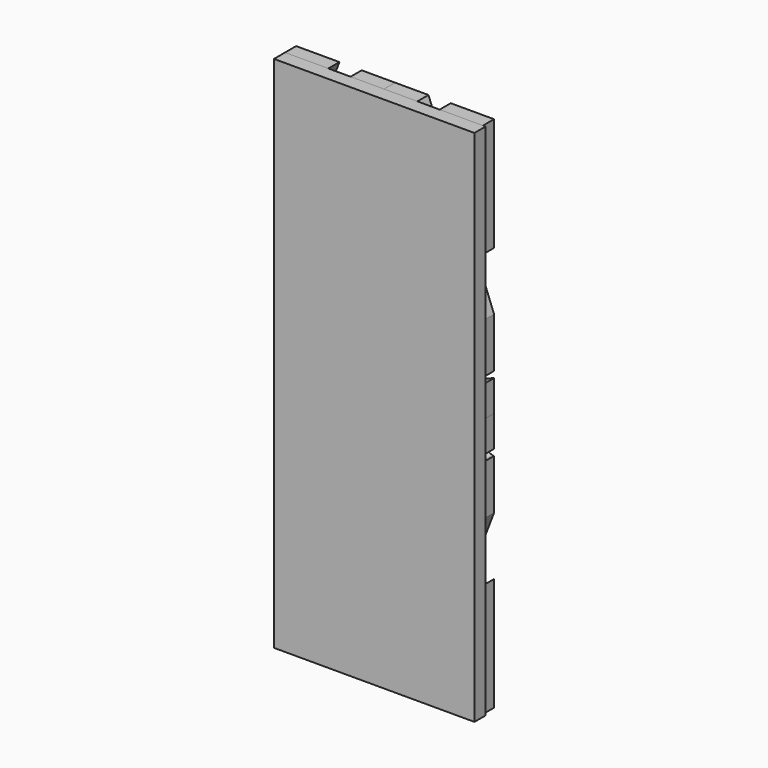
from build123d import *

# Parameters (mm, degrees)
F1_DEPTH = 2.54
F2_W     = 36.7250956763
F2_H     = 94.9781656687
F3_DEPTH = 2.54


with BuildPart() as f1:
    # F0 (on Front) → F1 (new body)
    with BuildSketch(Plane.XZ):
        Polygon((-10.1961911618, 47.455956084), (-18.1265615095, 47.455956084), (-18.1265615095, 26.6939761161), align=None)
    extrude(amount=F1_DEPTH)


with BuildPart() as f1b:
    # F0 (on Front) → F1, piece 2 (new body)
    with BuildSketch(Plane.XZ):
        Polygon((-3.3987303873, 47.455956084), (-6.1177146971, 47.455956084), (-18.1265615095, 16.0163856696), (-18.1265615095, 8.8979920387), align=None)
        with BuildLine():
            Line((0, 47.455956084), (-3.3987303873, 47.455956084))
            Line((-3.3987303873, 47.455956084), (-18.1265615095, 8.8979920387))
            Line((-18.1265615095, 8.8979920387), (-18.1265615095, 6.8514491871))
            ThreePointArc((-18.1265615095, 6.8514491871), (-17.9774288105, 6.8556010302), (-17.8323030506, 6.8210132649))
            Line((-17.8323030506, 6.8210132649), (-15.815424917, 6.0506344007))
            Line((-15.815424917, 6.0506344007), (-14.6774796667, 9.029813866))
            Line((-14.6774796667, 9.029813866), (-16.6943578003, 9.8001927301))
            ThreePointArc((-16.6943578003, 9.8001927301), (-17.0243134892, 10.5379960531), (-16.2865101663, 10.867951742))
            Line((-16.2865101663, 10.867951742), (-14.2696320327, 10.0975728779))
            Line((-14.2696320327, 10.0975728779), (-13.1316867824, 13.0767523431))
            Line((-13.1316867824, 13.0767523431), (-15.148564916, 13.8471312073))
            ThreePointArc((-15.148564916, 13.8471312073), (-15.478520605, 14.5849345302), (-14.740717282, 14.9148902192))
            Line((-14.740717282, 14.9148902192), (-12.7238391485, 14.144511355))
            Line((-12.7238391485, 14.144511355), (-11.5858938981, 17.1236908203))
            Line((-11.5858938981, 17.1236908203), (-13.6027720317, 17.8940696845))
            ThreePointArc((-13.6027720317, 17.8940696845), (-13.9327277207, 18.6318730074), (-13.1949243977, 18.9618286963))
            Line((-13.1949243977, 18.9618286963), (-11.1780462642, 18.1914498322))
            Line((-11.1780462642, 18.1914498322), (-10.0401010139, 21.1706292975))
            Line((-10.0401010139, 21.1706292975), (-12.0569791474, 21.9410081616))
            ThreePointArc((-12.0569791474, 21.9410081616), (-12.3869348364, 22.6788114845), (-11.6491315135, 23.0087671735))
            Line((-11.6491315135, 23.0087671735), (-9.6322533799, 22.2383883093))
            Line((-9.6322533799, 22.2383883093), (-9.0632807547, 23.727978042))
            Line((-9.0632807547, 23.727978042), (-8.4943081296, 25.2175677746))
            Line((-8.4943081296, 25.2175677746), (-10.5111862631, 25.9879466388))
            ThreePointArc((-10.5111862631, 25.9879466388), (-10.8411419521, 26.7257499617), (-10.1033386292, 27.0557056507))
            Line((-10.1033386292, 27.0557056507), (-8.0864604956, 26.2853267865))
            Line((-8.0864604956, 26.2853267865), (-6.9485152453, 29.2645062518))
            Line((-6.9485152453, 29.2645062518), (-8.9653933789, 30.0348851159))
            ThreePointArc((-8.9653933789, 30.0348851159), (-9.2953490678, 30.7726884389), (-8.5575457449, 31.1026441278))
            Line((-8.5575457449, 31.1026441278), (-6.5406676113, 30.3322652637))
            Line((-6.5406676113, 30.3322652637), (-5.402722361, 33.3114447289))
            Line((-5.402722361, 33.3114447289), (-7.4196004946, 34.0818235931))
            ThreePointArc((-7.4196004946, 34.0818235931), (-7.7495561835, 34.819626916), (-7.0117528606, 35.149582605))
            Line((-7.0117528606, 35.149582605), (-4.9948747271, 34.3792037408))
            Line((-4.9948747271, 34.3792037408), (-3.8569294767, 37.3583832061))
            Line((-3.8569294767, 37.3583832061), (-5.8738076103, 38.1287620703))
            ThreePointArc((-5.8738076103, 38.1287620703), (-6.2037632993, 38.8665653932), (-5.4659599763, 39.1965210821))
            Line((-5.4659599763, 39.1965210821), (-3.4490818428, 38.426142218))
            Line((-3.4490818428, 38.426142218), (-2.3111365925, 41.4053216833))
            Line((-2.3111365925, 41.4053216833), (-4.328014726, 42.1757005474))
            ThreePointArc((-4.328014726, 42.1757005474), (-4.657970415, 42.9135038703), (-3.9201670921, 43.2434595593))
            Line((-3.9201670921, 43.2434595593), (-1.9032889585, 42.4730806951))
            Line((-1.9032889585, 42.4730806951), (0, 47.455956084))
        make_face()
    extrude(amount=F1_DEPTH)


with BuildPart() as f1c:
    # F0 (on Front) → F1, piece 3 (new body)
    with BuildSketch(Plane.XZ):
        with BuildLine():
            Line((3.3987303873, 47.455956084), (0, 47.455956084))
            Line((0, 47.455956084), (1.9032889585, 42.4730806951))
            Line((1.9032889585, 42.4730806951), (3.9201670921, 43.2434595593))
            ThreePointArc((3.9201670921, 43.2434595593), (4.657970415, 42.9135038703), (4.328014726, 42.1757005474))
            Line((4.328014726, 42.1757005474), (2.3111365925, 41.4053216833))
            Line((2.3111365925, 41.4053216833), (3.4490818428, 38.426142218))
            Line((3.4490818428, 38.426142218), (5.4659599763, 39.1965210821))
            ThreePointArc((5.4659599763, 39.1965210821), (6.2037632993, 38.8665653932), (5.8738076103, 38.1287620703))
            Line((5.8738076103, 38.1287620703), (3.8569294767, 37.3583832061))
            Line((3.8569294767, 37.3583832061), (4.9948747271, 34.3792037408))
            Line((4.9948747271, 34.3792037408), (7.0117528606, 35.149582605))
            ThreePointArc((7.0117528606, 35.149582605), (7.7495561835, 34.819626916), (7.4196004946, 34.0818235931))
            Line((7.4196004946, 34.0818235931), (5.402722361, 33.3114447289))
            Line((5.402722361, 33.3114447289), (6.5406676113, 30.3322652637))
            Line((6.5406676113, 30.3322652637), (8.5575457449, 31.1026441278))
            ThreePointArc((8.5575457449, 31.1026441278), (9.2953490678, 30.7726884389), (8.9653933789, 30.0348851159))
            Line((8.9653933789, 30.0348851159), (6.9485152453, 29.2645062518))
            Line((6.9485152453, 29.2645062518), (8.0864604956, 26.2853267865))
            Line((8.0864604956, 26.2853267865), (10.1033386292, 27.0557056507))
            ThreePointArc((10.1033386292, 27.0557056507), (10.8411419521, 26.7257499617), (10.5111862631, 25.9879466388))
            Line((10.5111862631, 25.9879466388), (8.4943081296, 25.2175677746))
            Line((8.4943081296, 25.2175677746), (9.6322533799, 22.2383883093))
            Line((9.6322533799, 22.2383883093), (11.6491315135, 23.0087671735))
            ThreePointArc((11.6491315135, 23.0087671735), (12.3869348364, 22.6788114845), (12.0569791474, 21.9410081616))
            Line((12.0569791474, 21.9410081616), (10.0401010139, 21.1706292975))
            Line((10.0401010139, 21.1706292975), (11.1780462642, 18.1914498322))
            Line((11.1780462642, 18.1914498322), (13.1949243977, 18.9618286963))
            ThreePointArc((13.1949243977, 18.9618286963), (13.9327277207, 18.6318730074), (13.6027720317, 17.8940696845))
            Line((13.6027720317, 17.8940696845), (11.5858938981, 17.1236908203))
            Line((11.5858938981, 17.1236908203), (12.7238391485, 14.144511355))
            Line((12.7238391485, 14.144511355), (14.740717282, 14.9148902192))
            ThreePointArc((14.740717282, 14.9148902192), (15.478520605, 14.5849345302), (15.148564916, 13.8471312073))
            Line((15.148564916, 13.8471312073), (13.1316867824, 13.0767523431))
            Line((13.1316867824, 13.0767523431), (14.2696320327, 10.0975728779))
            Line((14.2696320327, 10.0975728779), (16.2865101663, 10.867951742))
            ThreePointArc((16.2865101663, 10.867951742), (17.0243134892, 10.5379960531), (16.6943578003, 9.8001927301))
            Line((16.6943578003, 9.8001927301), (14.6774796667, 9.029813866))
            Line((14.6774796667, 9.029813866), (15.815424917, 6.0506344007))
            Line((15.815424917, 6.0506344007), (17.8323030506, 6.8210132649))
            ThreePointArc((17.8323030506, 6.8210132649), (17.9774288105, 6.8556010302), (18.1265615095, 6.8514491871))
            Line((18.1265615095, 6.8514491871), (18.1265615095, 8.8979920387))
            Line((18.1265615095, 8.8979920387), (3.3987303873, 47.455956084))
        make_face()
        Polygon((6.1177146971, 47.455956084), (3.3987303873, 47.455956084), (18.1265615095, 8.8979920387), (18.1265615095, 16.0163856696), align=None)
    extrude(amount=F1_DEPTH)


with BuildPart() as f1d:
    # F0 (on Front) → F1, piece 4 (new body)
    with BuildSketch(Plane.XZ):
        Polygon((-16.223272551, 4.9828753888), (-18.1265615095, 5.7098670506), (-18.1265615095, 0), align=None)
    extrude(amount=F1_DEPTH)


with BuildPart() as f1e:
    # F0 (on Front) → F1, piece 5 (new body)
    with BuildSketch(Plane.XZ):
        Polygon((18.1265615095, 47.455956084), (10.1961911618, 47.455956084), (18.1265615095, 26.6939761161), align=None)
    extrude(amount=F1_DEPTH)


with BuildPart() as f1f:
    # F0 (on Front) → F1, piece 6 (new body)
    with BuildSketch(Plane.XZ):
        Polygon((-16.223272551, -4.9828753888), (-18.1265615095, 0), (-18.1265615095, -5.7098670506), align=None)
    extrude(amount=F1_DEPTH)


with BuildPart() as f1g:
    # F0 (on Front) → F1, piece 7 (new body)
    with BuildSketch(Plane.XZ):
        Polygon((18.1265615095, 0), (18.1265615095, 5.7098670506), (16.223272551, 4.9828753888), align=None)
    extrude(amount=F1_DEPTH)


with BuildPart() as f1h:
    # F0 (on Front) → F1, piece 8 (new body)
    with BuildSketch(Plane.XZ):
        Polygon((18.1265615095, -5.7098670506), (18.1265615095, 0), (16.223272551, -4.9828753888), align=None)
    extrude(amount=F1_DEPTH)


with BuildPart() as f1i:
    # F0 (on Front) → F1, piece 9 (new body)
    with BuildSketch(Plane.XZ):
        with BuildLine():
            ThreePointArc((-17.8323030506, -6.8210132649), (-17.9774288105, -6.8556010302), (-18.1265615095, -6.8514491871))
            Line((-18.1265615095, -6.8514491871), (-18.1265615095, -8.8979920387))
            Line((-18.1265615095, -8.8979920387), (-3.3987303873, -47.455956084))
            Line((-3.3987303873, -47.455956084), (0, -47.455956084))
            Line((0, -47.455956084), (-1.9032889585, -42.4730806951))
            Line((-1.9032889585, -42.4730806951), (-3.9201670921, -43.2434595593))
            ThreePointArc((-3.9201670921, -43.2434595593), (-4.657970415, -42.9135038703), (-4.328014726, -42.1757005474))
            Line((-4.328014726, -42.1757005474), (-2.3111365925, -41.4053216833))
            Line((-2.3111365925, -41.4053216833), (-3.4490818428, -38.426142218))
            Line((-3.4490818428, -38.426142218), (-5.4659599763, -39.1965210821))
            ThreePointArc((-5.4659599763, -39.1965210821), (-6.2037632993, -38.8665653932), (-5.8738076103, -38.1287620703))
            Line((-5.8738076103, -38.1287620703), (-3.8569294767, -37.3583832061))
            Line((-3.8569294767, -37.3583832061), (-4.9948747271, -34.3792037408))
            Line((-4.9948747271, -34.3792037408), (-7.0117528606, -35.149582605))
            ThreePointArc((-7.0117528606, -35.149582605), (-7.7495561835, -34.819626916), (-7.4196004946, -34.0818235931))
            Line((-7.4196004946, -34.0818235931), (-5.402722361, -33.3114447289))
            Line((-5.402722361, -33.3114447289), (-6.5406676113, -30.3322652637))
            Line((-6.5406676113, -30.3322652637), (-8.5575457449, -31.1026441278))
            ThreePointArc((-8.5575457449, -31.1026441278), (-9.2953490678, -30.7726884389), (-8.9653933789, -30.0348851159))
            Line((-8.9653933789, -30.0348851159), (-6.9485152453, -29.2645062518))
            Line((-6.9485152453, -29.2645062518), (-8.0864604956, -26.2853267865))
            Line((-8.0864604956, -26.2853267865), (-10.1033386292, -27.0557056507))
            ThreePointArc((-10.1033386292, -27.0557056507), (-10.8411419521, -26.7257499617), (-10.5111862631, -25.9879466388))
            Line((-10.5111862631, -25.9879466388), (-8.4943081296, -25.2175677746))
            Line((-8.4943081296, -25.2175677746), (-9.6322533799, -22.2383883093))
            Line((-9.6322533799, -22.2383883093), (-11.6491315135, -23.0087671735))
            ThreePointArc((-11.6491315135, -23.0087671735), (-12.3869348364, -22.6788114845), (-12.0569791474, -21.9410081616))
            Line((-12.0569791474, -21.9410081616), (-10.0401010139, -21.1706292975))
            Line((-10.0401010139, -21.1706292975), (-11.1780462642, -18.1914498322))
            Line((-11.1780462642, -18.1914498322), (-13.1949243977, -18.9618286963))
            ThreePointArc((-13.1949243977, -18.9618286963), (-13.9327277207, -18.6318730074), (-13.6027720317, -17.8940696845))
            Line((-13.6027720317, -17.8940696845), (-11.5858938981, -17.1236908203))
            Line((-11.5858938981, -17.1236908203), (-12.7238391485, -14.144511355))
            Line((-12.7238391485, -14.144511355), (-14.740717282, -14.9148902192))
            ThreePointArc((-14.740717282, -14.9148902192), (-15.478520605, -14.5849345302), (-15.148564916, -13.8471312073))
            Line((-15.148564916, -13.8471312073), (-13.1316867824, -13.0767523431))
            Line((-13.1316867824, -13.0767523431), (-14.2696320327, -10.0975728779))
            Line((-14.2696320327, -10.0975728779), (-16.2865101663, -10.867951742))
            ThreePointArc((-16.2865101663, -10.867951742), (-17.0243134892, -10.5379960531), (-16.6943578003, -9.8001927301))
            Line((-16.6943578003, -9.8001927301), (-14.6774796667, -9.029813866))
            Line((-14.6774796667, -9.029813866), (-15.815424917, -6.0506344007))
            Line((-15.815424917, -6.0506344007), (-17.8323030506, -6.8210132649))
        make_face()
        Polygon((-3.3987303873, -47.455956084), (-18.1265615095, -8.8979920387), (-18.1265615095, -16.0163856696), (-6.1177146971, -47.455956084), align=None)
    extrude(amount=F1_DEPTH)


with BuildPart() as f1j:
    # F0 (on Front) → F1, piece 10 (new body)
    with BuildSketch(Plane.XZ):
        with BuildLine():
            Line((18.1265615095, -8.8979920387), (18.1265615095, -6.8514491871))
            ThreePointArc((18.1265615095, -6.8514491871), (17.9774288105, -6.8556010302), (17.8323030506, -6.8210132649))
            Line((17.8323030506, -6.8210132649), (15.815424917, -6.0506344007))
            Line((15.815424917, -6.0506344007), (14.6774796667, -9.029813866))
            Line((14.6774796667, -9.029813866), (16.6943578003, -9.8001927301))
            ThreePointArc((16.6943578003, -9.8001927301), (17.0243134892, -10.5379960531), (16.2865101663, -10.867951742))
            Line((16.2865101663, -10.867951742), (14.2696320327, -10.0975728779))
            Line((14.2696320327, -10.0975728779), (13.1316867824, -13.0767523431))
            Line((13.1316867824, -13.0767523431), (15.148564916, -13.8471312073))
            ThreePointArc((15.148564916, -13.8471312073), (15.478520605, -14.5849345302), (14.740717282, -14.9148902192))
            Line((14.740717282, -14.9148902192), (12.7238391485, -14.144511355))
            Line((12.7238391485, -14.144511355), (11.5858938981, -17.1236908203))
            Line((11.5858938981, -17.1236908203), (13.6027720317, -17.8940696845))
            ThreePointArc((13.6027720317, -17.8940696845), (13.9327277207, -18.6318730074), (13.1949243977, -18.9618286963))
            Line((13.1949243977, -18.9618286963), (11.1780462642, -18.1914498322))
            Line((11.1780462642, -18.1914498322), (10.0401010139, -21.1706292975))
            Line((10.0401010139, -21.1706292975), (12.0569791474, -21.9410081616))
            ThreePointArc((12.0569791474, -21.9410081616), (12.3869348364, -22.6788114845), (11.6491315135, -23.0087671735))
            Line((11.6491315135, -23.0087671735), (9.6322533799, -22.2383883093))
            Line((9.6322533799, -22.2383883093), (8.4943081296, -25.2175677746))
            Line((8.4943081296, -25.2175677746), (10.5111862631, -25.9879466388))
            ThreePointArc((10.5111862631, -25.9879466388), (10.8411419521, -26.7257499617), (10.1033386292, -27.0557056507))
            Line((10.1033386292, -27.0557056507), (8.0864604956, -26.2853267865))
            Line((8.0864604956, -26.2853267865), (6.9485152453, -29.2645062518))
            Line((6.9485152453, -29.2645062518), (8.9653933789, -30.0348851159))
            ThreePointArc((8.9653933789, -30.0348851159), (9.2953490678, -30.7726884389), (8.5575457449, -31.1026441278))
            Line((8.5575457449, -31.1026441278), (6.5406676113, -30.3322652637))
            Line((6.5406676113, -30.3322652637), (5.402722361, -33.3114447289))
            Line((5.402722361, -33.3114447289), (7.4196004946, -34.0818235931))
            ThreePointArc((7.4196004946, -34.0818235931), (7.7495561835, -34.819626916), (7.0117528606, -35.149582605))
            Line((7.0117528606, -35.149582605), (4.9948747271, -34.3792037408))
            Line((4.9948747271, -34.3792037408), (3.8569294767, -37.3583832061))
            Line((3.8569294767, -37.3583832061), (5.8738076103, -38.1287620703))
            ThreePointArc((5.8738076103, -38.1287620703), (6.2037632993, -38.8665653932), (5.4659599763, -39.1965210821))
            Line((5.4659599763, -39.1965210821), (3.4490818428, -38.426142218))
            Line((3.4490818428, -38.426142218), (2.3111365925, -41.4053216833))
            Line((2.3111365925, -41.4053216833), (4.328014726, -42.1757005474))
            ThreePointArc((4.328014726, -42.1757005474), (4.657970415, -42.9135038703), (3.9201670921, -43.2434595593))
            Line((3.9201670921, -43.2434595593), (1.9032889585, -42.4730806951))
            Line((1.9032889585, -42.4730806951), (0, -47.455956084))
            Line((0, -47.455956084), (3.3987303873, -47.455956084))
            Line((3.3987303873, -47.455956084), (18.1265615095, -8.8979920387))
        make_face()
        Polygon((18.1265615095, -16.0163856696), (18.1265615095, -8.8979920387), (3.3987303873, -47.455956084), (6.1177146971, -47.455956084), align=None)
    extrude(amount=F1_DEPTH)


with BuildPart() as f1k:
    # F0 (on Front) → F1, piece 11 (new body)
    with BuildSketch(Plane.XZ):
        Polygon((-10.1961911618, -47.455956084), (-18.1265615095, -26.6939761161), (-18.1265615095, -47.455956084), align=None)
    extrude(amount=F1_DEPTH)


with BuildPart() as f1l:
    # F0 (on Front) → F1, piece 12 (new body)
    with BuildSketch(Plane.XZ):
        Polygon((18.1265615095, -47.455956084), (18.1265615095, -26.6939761161), (10.1961911618, -47.455956084), align=None)
    extrude(amount=F1_DEPTH)


with BuildPart() as f1m:
    # F0 (on Front) → F1, piece 13 (new body)
    with BuildSketch(Plane.XZ):
        with BuildLine():
            Line((0.3851894321, 28.6515334857), (0, 29.6599725525))
            Line((0, 29.6599725525), (-0.3851894321, 28.6515334857))
            Line((-0.3851894321, 28.6515334857), (-2.4020675656, 29.4219123498))
            ThreePointArc((-2.4020675656, 29.4219123498), (-3.1398708886, 29.0919566609), (-2.8099151996, 28.354153338))
            Line((-2.8099151996, 28.354153338), (-0.793037066, 27.5837744738))
            Line((-0.793037066, 27.5837744738), (-1.8353143528, 24.855056999))
            Line((-1.8353143528, 24.855056999), (-3.8521924864, 25.6254358631))
            ThreePointArc((-3.8521924864, 25.6254358631), (-4.5899958093, 25.2954801742), (-4.2600401204, 24.5576768512))
            Line((-4.2600401204, 24.5576768512), (-2.2431619868, 23.7872979871))
            Line((-2.2431619868, 23.7872979871), (-3.2854392736, 21.0585805123))
            Line((-3.2854392736, 21.0585805123), (-5.3023174072, 21.8289593764))
            ThreePointArc((-5.3023174072, 21.8289593764), (-6.0401207301, 21.4990036874), (-5.7101650411, 20.7612003645))
            Line((-5.7101650411, 20.7612003645), (-3.6932869076, 19.9908215004))
            Line((-3.6932869076, 19.9908215004), (-4.7355641943, 17.2621040255))
            Line((-4.7355641943, 17.2621040255), (-6.7524423279, 18.0324828897))
            ThreePointArc((-6.7524423279, 18.0324828897), (-7.4902456508, 17.7025272007), (-7.1602899619, 16.9647238778))
            Line((-7.1602899619, 16.9647238778), (-5.1434118283, 16.1943450137))
            Line((-5.1434118283, 16.1943450137), (-6.1856891151, 13.4656275388))
            Line((-6.1856891151, 13.4656275388), (-8.2025672487, 14.236006403))
            ThreePointArc((-8.2025672487, 14.236006403), (-8.9403705716, 13.906050714), (-8.6104148826, 13.1682473911))
            Line((-8.6104148826, 13.1682473911), (-6.5935367491, 12.3978685269))
            Line((-6.5935367491, 12.3978685269), (-7.6358140359, 9.6691510521))
            Line((-7.6358140359, 9.6691510521), (-9.6526921694, 10.4395299163))
            ThreePointArc((-9.6526921694, 10.4395299163), (-10.3904954924, 10.1095742273), (-10.0605398034, 9.3717709044))
            Line((-10.0605398034, 9.3717709044), (-8.0436616698, 8.6013920402))
            Line((-8.0436616698, 8.6013920402), (-9.0859389566, 5.8726745654))
            Line((-9.0859389566, 5.8726745654), (-11.1028170902, 6.6430534295))
            ThreePointArc((-11.1028170902, 6.6430534295), (-11.8406204131, 6.3130977406), (-11.5106647242, 5.5752944177))
            Line((-11.5106647242, 5.5752944177), (-9.4937865906, 4.8049155535))
            Line((-9.4937865906, 4.8049155535), (-10.5360638774, 2.0761980787))
            Line((-10.5360638774, 2.0761980787), (-12.5529420109, 2.8465769428))
            Line((-12.5529420109, 2.8465769428), (-12.9607896449, 1.7788179309))
            Line((-12.9607896449, 1.7788179309), (-10.9439115113, 1.0084390668))
            Line((-10.9439115113, 1.0084390668), (-11.3291009434, 0))
            Line((-11.3291009434, 0), (-10.9439115113, -1.0084390668))
            Line((-10.9439115113, -1.0084390668), (-12.9607896449, -1.7788179309))
            Line((-12.9607896449, -1.7788179309), (-12.5529420109, -2.8465769428))
            Line((-12.5529420109, -2.8465769428), (-10.5360638774, -2.0761980787))
            Line((-10.5360638774, -2.0761980787), (-9.4937865906, -4.8049155535))
            Line((-9.4937865906, -4.8049155535), (-11.5106647242, -5.5752944177))
            ThreePointArc((-11.5106647242, -5.5752944177), (-11.8406204131, -6.3130977406), (-11.1028170902, -6.6430534295))
            Line((-11.1028170902, -6.6430534295), (-9.0859389566, -5.8726745654))
            Line((-9.0859389566, -5.8726745654), (-8.0436616698, -8.6013920402))
            Line((-8.0436616698, -8.6013920402), (-10.0605398034, -9.3717709044))
            ThreePointArc((-10.0605398034, -9.3717709044), (-10.3904954924, -10.1095742273), (-9.6526921694, -10.4395299163))
            Line((-9.6526921694, -10.4395299163), (-7.6358140359, -9.6691510521))
            Line((-7.6358140359, -9.6691510521), (-6.5935367491, -12.3978685269))
            Line((-6.5935367491, -12.3978685269), (-8.6104148826, -13.1682473911))
            ThreePointArc((-8.6104148826, -13.1682473911), (-8.9403705716, -13.906050714), (-8.2025672487, -14.236006403))
            Line((-8.2025672487, -14.236006403), (-6.1856891151, -13.4656275388))
            Line((-6.1856891151, -13.4656275388), (-5.1434118283, -16.1943450137))
            Line((-5.1434118283, -16.1943450137), (-7.1602899619, -16.9647238778))
            ThreePointArc((-7.1602899619, -16.9647238778), (-7.4902456508, -17.7025272007), (-6.7524423279, -18.0324828897))
            Line((-6.7524423279, -18.0324828897), (-4.7355641943, -17.2621040255))
            Line((-4.7355641943, -17.2621040255), (-3.6932869076, -19.9908215004))
            Line((-3.6932869076, -19.9908215004), (-5.7101650411, -20.7612003645))
            ThreePointArc((-5.7101650411, -20.7612003645), (-6.0401207301, -21.4990036874), (-5.3023174072, -21.8289593764))
            Line((-5.3023174072, -21.8289593764), (-3.2854392736, -21.0585805123))
            Line((-3.2854392736, -21.0585805123), (-2.2431619868, -23.7872979871))
            Line((-2.2431619868, -23.7872979871), (-4.2600401204, -24.5576768512))
            ThreePointArc((-4.2600401204, -24.5576768512), (-4.5899958093, -25.2954801742), (-3.8521924864, -25.6254358631))
            Line((-3.8521924864, -25.6254358631), (-1.8353143528, -24.855056999))
            Line((-1.8353143528, -24.855056999), (-0.793037066, -27.5837744738))
            Line((-0.793037066, -27.5837744738), (-2.8099151996, -28.354153338))
            ThreePointArc((-2.8099151996, -28.354153338), (-3.1398708886, -29.0919566609), (-2.4020675656, -29.4219123498))
            Line((-2.4020675656, -29.4219123498), (-0.3851894321, -28.6515334857))
            Line((-0.3851894321, -28.6515334857), (0, -29.6599725525))
            Line((0, -29.6599725525), (0.3851894321, -28.6515334857))
            Line((0.3851894321, -28.6515334857), (2.4020675656, -29.4219123498))
            ThreePointArc((2.4020675656, -29.4219123498), (3.1398708886, -29.0919566609), (2.8099151996, -28.354153338))
            Line((2.8099151996, -28.354153338), (0.793037066, -27.5837744738))
            Line((0.793037066, -27.5837744738), (1.8353143528, -24.855056999))
            Line((1.8353143528, -24.855056999), (3.8521924864, -25.6254358631))
            ThreePointArc((3.8521924864, -25.6254358631), (4.5899958093, -25.2954801742), (4.2600401204, -24.5576768512))
            Line((4.2600401204, -24.5576768512), (2.2431619868, -23.7872979871))
            Line((2.2431619868, -23.7872979871), (3.2854392736, -21.0585805123))
            Line((3.2854392736, -21.0585805123), (5.3023174072, -21.8289593764))
            ThreePointArc((5.3023174072, -21.8289593764), (6.0401207301, -21.4990036874), (5.7101650411, -20.7612003645))
            Line((5.7101650411, -20.7612003645), (3.6932869076, -19.9908215004))
            Line((3.6932869076, -19.9908215004), (4.7355641943, -17.2621040255))
            Line((4.7355641943, -17.2621040255), (6.7524423279, -18.0324828897))
            ThreePointArc((6.7524423279, -18.0324828897), (7.4902456508, -17.7025272007), (7.1602899619, -16.9647238778))
            Line((7.1602899619, -16.9647238778), (5.1434118283, -16.1943450137))
            Line((5.1434118283, -16.1943450137), (6.1856891151, -13.4656275388))
            Line((6.1856891151, -13.4656275388), (8.2025672487, -14.236006403))
            ThreePointArc((8.2025672487, -14.236006403), (8.9403705716, -13.906050714), (8.6104148826, -13.1682473911))
            Line((8.6104148826, -13.1682473911), (6.5935367491, -12.3978685269))
            Line((6.5935367491, -12.3978685269), (7.6358140359, -9.6691510521))
            Line((7.6358140359, -9.6691510521), (9.6526921694, -10.4395299163))
            ThreePointArc((9.6526921694, -10.4395299163), (10.3904954924, -10.1095742273), (10.0605398034, -9.3717709044))
            Line((10.0605398034, -9.3717709044), (8.0436616698, -8.6013920402))
            Line((8.0436616698, -8.6013920402), (9.0859389566, -5.8726745654))
            Line((9.0859389566, -5.8726745654), (11.1028170902, -6.6430534295))
            ThreePointArc((11.1028170902, -6.6430534295), (11.8406204131, -6.3130977406), (11.5106647242, -5.5752944177))
            Line((11.5106647242, -5.5752944177), (9.4937865906, -4.8049155535))
            Line((9.4937865906, -4.8049155535), (10.5360638774, -2.0761980787))
            Line((10.5360638774, -2.0761980787), (12.5529420109, -2.8465769428))
            Line((12.5529420109, -2.8465769428), (12.9607896449, -1.7788179309))
            Line((12.9607896449, -1.7788179309), (10.9439115113, -1.0084390668))
            Line((10.9439115113, -1.0084390668), (11.3291009434, 0))
            Line((11.3291009434, 0), (10.9439115113, 1.0084390668))
            Line((10.9439115113, 1.0084390668), (12.9607896449, 1.7788179309))
            ThreePointArc((12.9607896449, 1.7788179309), (13.2907453339, 2.5166212539), (12.552942011, 2.8465769428))
            Line((12.552942011, 2.8465769428), (10.5360638774, 2.0761980787))
            Line((10.5360638774, 2.0761980787), (9.4937865906, 4.8049155535))
            Line((9.4937865906, 4.8049155535), (11.5106647242, 5.5752944177))
            ThreePointArc((11.5106647242, 5.5752944177), (11.8406204131, 6.3130977406), (11.1028170902, 6.6430534295))
            Line((11.1028170902, 6.6430534295), (9.0859389566, 5.8726745654))
            Line((9.0859389566, 5.8726745654), (8.0436616698, 8.6013920402))
            Line((8.0436616698, 8.6013920402), (10.0605398034, 9.3717709044))
            ThreePointArc((10.0605398034, 9.3717709044), (10.3904954924, 10.1095742273), (9.6526921694, 10.4395299163))
            Line((9.6526921694, 10.4395299163), (7.6358140359, 9.6691510521))
            Line((7.6358140359, 9.6691510521), (6.5935367491, 12.3978685269))
            Line((6.5935367491, 12.3978685269), (8.6104148826, 13.1682473911))
            ThreePointArc((8.6104148826, 13.1682473911), (8.9403705716, 13.906050714), (8.2025672487, 14.236006403))
            Line((8.2025672487, 14.236006403), (6.1856891151, 13.4656275388))
            Line((6.1856891151, 13.4656275388), (5.1434118283, 16.1943450137))
            Line((5.1434118283, 16.1943450137), (7.1602899619, 16.9647238778))
            ThreePointArc((7.1602899619, 16.9647238778), (7.4902456508, 17.7025272007), (6.7524423279, 18.0324828897))
            Line((6.7524423279, 18.0324828897), (4.7355641943, 17.2621040255))
            Line((4.7355641943, 17.2621040255), (3.6932869076, 19.9908215004))
            Line((3.6932869076, 19.9908215004), (5.7101650411, 20.7612003645))
            ThreePointArc((5.7101650411, 20.7612003645), (6.0401207301, 21.4990036874), (5.3023174072, 21.8289593764))
            Line((5.3023174072, 21.8289593764), (3.2854392736, 21.0585805123))
            Line((3.2854392736, 21.0585805123), (2.2431619868, 23.7872979871))
            Line((2.2431619868, 23.7872979871), (4.2600401204, 24.5576768512))
            ThreePointArc((4.2600401204, 24.5576768512), (4.5899958093, 25.2954801742), (3.8521924864, 25.6254358631))
            Line((3.8521924864, 25.6254358631), (1.8353143528, 24.855056999))
            Line((1.8353143528, 24.855056999), (0.793037066, 27.5837744738))
            Line((0.793037066, 27.5837744738), (2.8099151996, 28.354153338))
            Line((2.8099151996, 28.354153338), (2.4020675656, 29.4219123498))
            Line((2.4020675656, 29.4219123498), (0.3851894321, 28.6515334857))
        make_face()
        Polygon((-7.9303705561, 0), (0, 20.7619805138), (7.9303705561, 0), (0, -20.7619805138), align=None, mode=Mode.SUBTRACT)
        with BuildLine():
            Line((-12.9607896449, 1.7788179309), (-12.5529420109, 2.8465769428))
            ThreePointArc((-12.5529420109, 2.8465769428), (-13.2907453339, 2.5166212539), (-12.9607896449, 1.7788179309))
        make_face()
        with BuildLine():
            Line((-12.5529420109, -2.8465769428), (-12.9607896449, -1.7788179309))
            ThreePointArc((-12.9607896449, -1.7788179309), (-13.2907453339, -2.5166212539), (-12.5529420109, -2.8465769428))
        make_face()
        with BuildLine():
            ThreePointArc((12.5529420109, -2.8465769428), (13.2907453339, -2.5166212539), (12.9607896449, -1.7788179309))
            Line((12.9607896449, -1.7788179309), (12.5529420109, -2.8465769428))
        make_face()
    extrude(amount=F1_DEPTH)


with BuildPart() as f1n:
    # F0 (on Front) → F1, piece 14 (new body)
    with BuildSketch(Plane.XZ):
        Polygon((0, -11.8639888323), (4.5316403053, 0), (0, 11.8639888323), (-4.5316403053, 0), align=None)
    extrude(amount=F1_DEPTH)


with BuildPart() as f3:
    # F2 (on face) → F3 (new body)
    with BuildSketch(Plane.XZ.offset(2.54)):
        with Locations((0.2359863287, -0.0331267504)):
            Rectangle(F2_W, F2_H)
    extrude(amount=F3_DEPTH)


solid = Compound([f1.part, f1b.part, f1c.part, f1d.part, f1e.part, f1f.part, f1g.part, f1h.part, f1i.part, f1j.part, f1k.part, f1l.part, f1m.part, f1n.part, f3.part])
